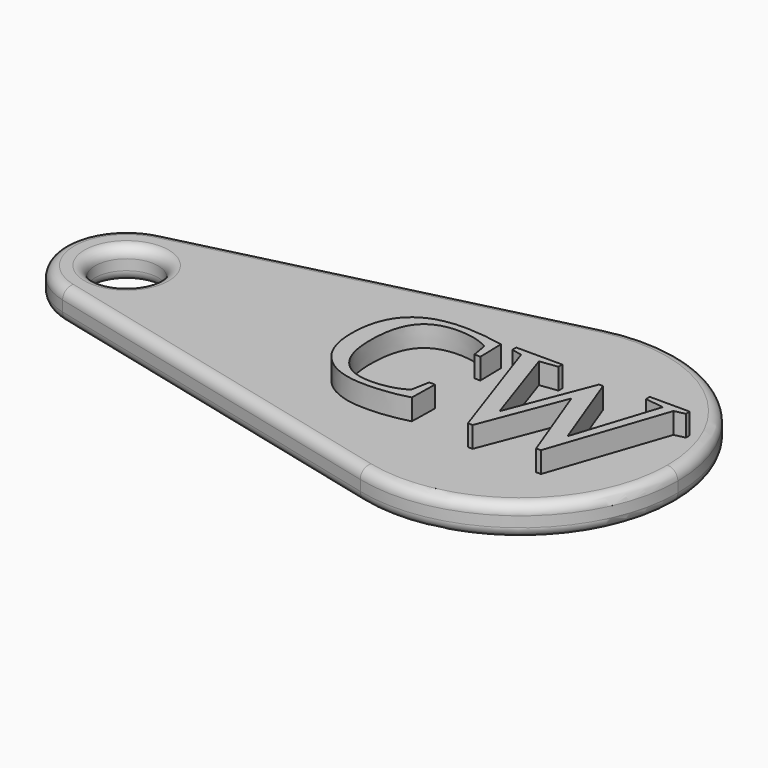
from build123d import *

# Parameters (mm, degrees)
F1_DEPTH     = 3
F2_R         = 3
F3_DEPTH     = 25
F4_TEXT_SIZE = 17.5627353233
F5_DEPTH     = 2
F6_R         = 1


# Not quite as in the source:
# - Text() gives the source's letters only with a copy of the font that has no kerning and outlines rounded to 1/6400 em; it was checked with that copy


with BuildPart() as f1:
    # F0 (on Top) → F1 (new body)
    with BuildSketch(Plane.XY):
        with BuildLine():
            ThreePointArc((14.9634298243, 0), (12.662078226, 4.7244047244), (7.5234298243, 5.8246373278))
            ThreePointArc((7.5234298243, 5.8246373278), (2.9634298243, 0), (7.5234298243, -5.8246373278))
            ThreePointArc((7.5234298243, -5.8246373278), (12.662078226, -4.7244047244), (14.9634298243, 0))
        make_face()
        with BuildLine():
            ThreePointArc((42.8634298243, -14.5615933194), (31.4634298243, 0), (42.8634298243, 14.5615933194))
            Line((42.8634298243, 14.5615933194), (7.5234298243, 5.8246373278))
            ThreePointArc((7.5234298243, 5.8246373278), (12.662078226, 4.7244047244), (14.9634298243, 0))
            ThreePointArc((14.9634298243, 0), (12.662078226, -4.7244047244), (7.5234298243, -5.8246373278))
            Line((7.5234298243, -5.8246373278), (42.8634298243, -14.5615933194))
        make_face()
        with BuildLine():
            ThreePointArc((42.8634298243, -14.5615933194), (55.7100508287, -11.811011811), (61.4634298243, 0))
            ThreePointArc((61.4634298243, 0), (55.7100508287, 11.811011811), (42.8634298243, 14.5615933194))
            ThreePointArc((42.8634298243, 14.5615933194), (31.4634298243, 0), (42.8634298243, -14.5615933194))
        make_face()
    extrude(amount=F1_DEPTH)

    # F2 (on face) → F3 (cut)
    with BuildSketch(Plane.XY.offset(3)):
        with Locations((8.9634298243, 0)):
            Circle(F2_R)
    extrude(amount=-F3_DEPTH, mode=Mode.SUBTRACT)

    # F4 (on face) → F5 (join)
    with BuildSketch(Plane.XY.offset(3)):
        with Locations((30.5174719252, -6.7239810822)):
            Text('CW', F4_TEXT_SIZE, font='Tinos', text_align=(TextAlign.LEFT, TextAlign.BOTTOM))
    extrude(amount=F5_DEPTH)

    # F6
    f6_edges = [f1.edges().sort_by_distance(p)[0] for p in [
        (5.96343, 0, 3),
        (25.19343, -10.193115, 3),
        (25.19343, 10.193115, 0),
        (5.96343, 0, 0),
    ]]
    fillet(f6_edges, radius=F6_R)


solid = f1.part
